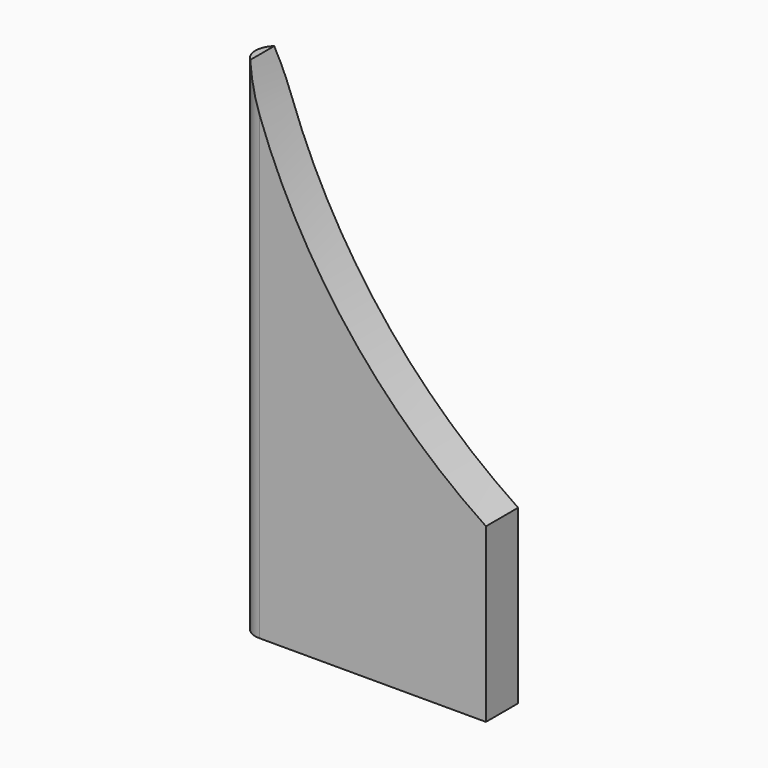
from build123d import *

# Parameters (mm, degrees)
F1_DEPTH = 12
F2_R     = 5.99999


# Not quite as in the source:
# - a fillet or chamfer is up to 0.001 mm smaller than in the source, because OpenCascade refuses the exact size


with BuildPart() as f1:
    # F0 (on Front) → F1 (new body)
    with BuildSketch(Plane.XZ):
        with BuildLine():
            Line((-118, -20.6604213454), (-44.4413209303, -20.6604213454))
            Line((-44.4413209303, -20.6604213454), (-44.4413209303, 30.7246802683))
            ThreePointArc((-44.4413209303, 30.7246802683), (-89.0802193772, 73.6033003164), (-116, 129.3395786546))
            Line((-116, 129.3395786546), (-118, 129.3395786546))
            Line((-118, 129.3395786546), (-118, -20.6604213454))
        make_face()
    extrude(amount=F1_DEPTH)

    # F2 (radius 6 in the source; OpenCascade refuses exactly that, so slightly less here)
    f2_edges = [f1.edges().sort_by_distance(p)[0] for p in [
        (-118, 0, 54.339579),
        (-118, -12, 54.339579),
    ]]
    fillet(f2_edges, radius=F2_R)


solid = f1.part
